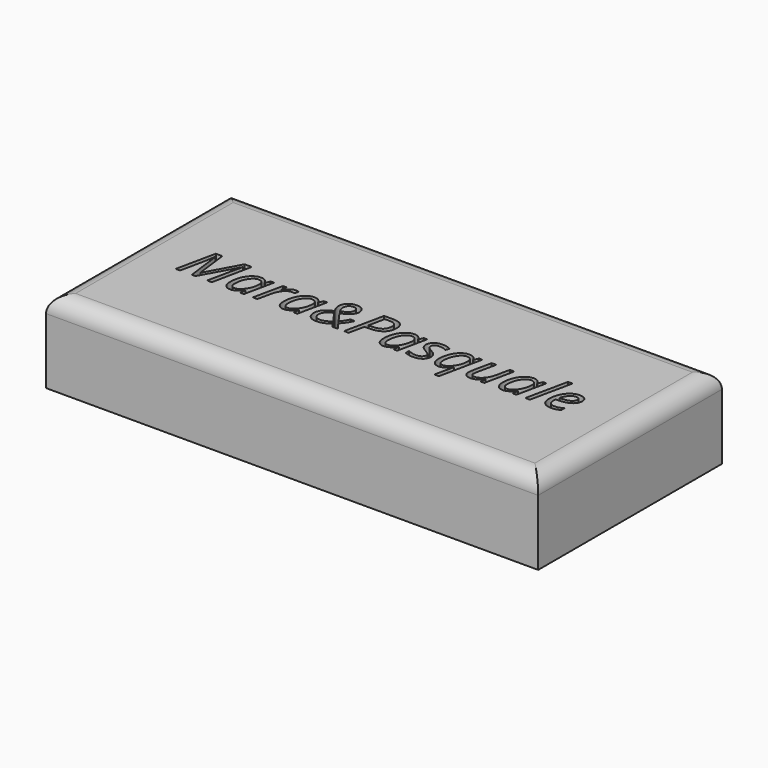
from build123d import *

# Parameters (mm, degrees)
F0_W         = 150
F0_H         = 70
F1_DEPTH     = 25
F2_TEXT_SIZE = 16.9177901137
F3_DEPTH     = 20
F4_R         = 5


# Not quite as in the source:
# - Text() gives the source's letters only with a copy of the font that has no kerning and outlines rounded to 1/6400 em; it was checked with that copy


with BuildPart() as f1:
    # F0 (on Top) → F1 (new body)
    with BuildSketch(Plane.XY):
        Rectangle(F0_W, F0_H)
    extrude(amount=F1_DEPTH)

    # F2 (on face) → F3 (cut)
    with BuildSketch(Plane.XY.offset(25)):
        with Locations((-60, -5.2326009288)):
            Text('Mara&Pasquale', F2_TEXT_SIZE, font='Open Sans', font_style=FontStyle.ITALIC, text_align=(TextAlign.LEFT, TextAlign.BOTTOM))
    extrude(amount=-F3_DEPTH, mode=Mode.SUBTRACT)

    # F4
    f4_edges = [f1.edges().sort_by_distance(p)[0] for p in [
        (-75, 0, 25),
        (0, 35, 25),
        (75, 0, 25),
        (0, -35, 25),
    ]]
    fillet(f4_edges, radius=F4_R)


solid = f1.part
